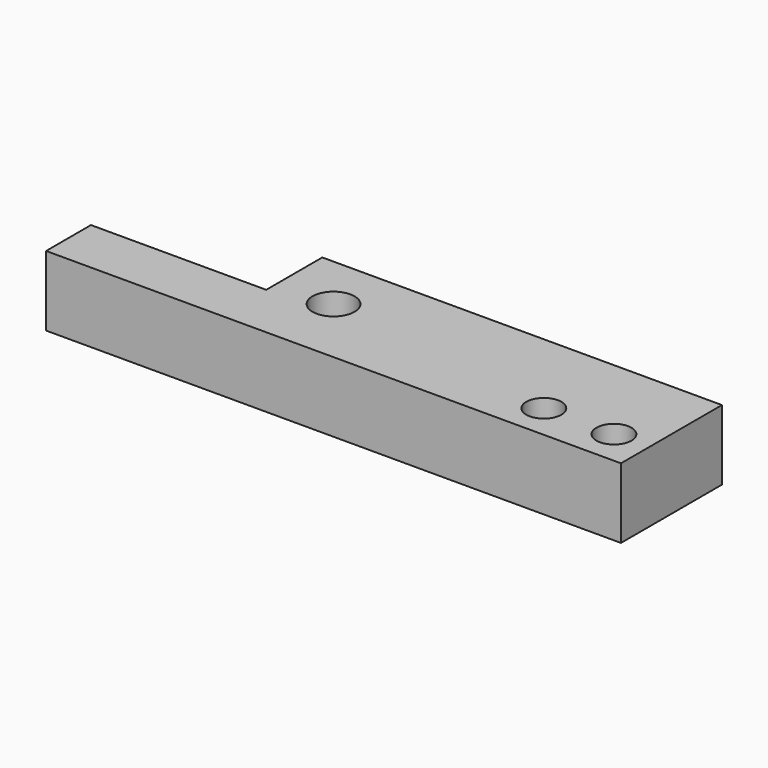
from build123d import *

# Parameters (mm, degrees)
F0_W     = 82
F0_H     = 20
F0_R     = 2.5
F0_R_2   = 3
F1_DEPTH = 10
F2_W     = 57
F2_H     = 2
F3_DEPTH = 10


# Not quite as in the source:
# - a feature names something its author has since deleted; it is built from what else it names


with BuildPart() as f1:
    # F0 (on Top) → F1 (new body)
    with BuildSketch(Plane.XY):
        Rectangle(F0_W, F0_H)
        with Locations((26, -5)):
            Circle(F0_R, mode=Mode.SUBTRACT)
        with Locations((36, -5)):
            Circle(F0_R, mode=Mode.SUBTRACT)
        with Locations((-8, 0)):
            Circle(F0_R_2, mode=Mode.SUBTRACT)
    extrude(amount=F1_DEPTH)

    # F2 (on face) → F3 (cut)
    with BuildSketch(Plane.XY.offset(10)):
        Polygon((-16, 10), (-41, 10), (-41, -2), (-16, -2), (-16, 8), align=None)
        with Locations((12.5, 9)):
            Rectangle(F2_W, F2_H)
    extrude(amount=-F3_DEPTH, mode=Mode.SUBTRACT)


solid = f1.part
